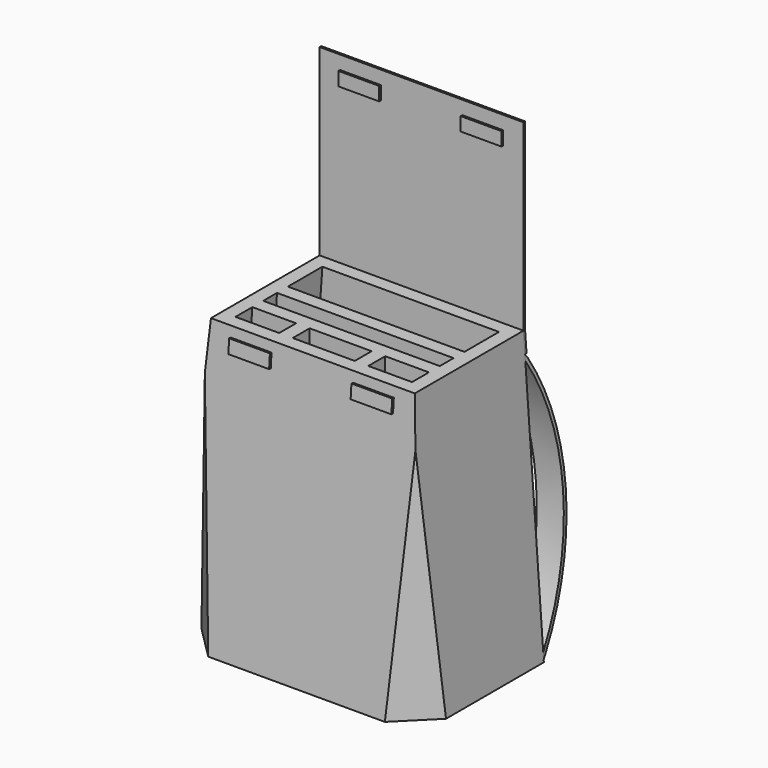
from build123d import *

# Parameters (mm, degrees)
F0_W      = 300
F0_H      = 200
F1_DEPTH  = 420
F3_DEPTH  = 420
F5_DEPTH  = 360
F7_DEPTH  = 230.001
F9_DEPTH  = 1000
F10_T     = -20
F11_W     = 317.0409461497
F11_H     = 20
F12_DEPTH = 400
F13_DEPTH = 25
F14_DEPTH = 25
F15_DEPTH = 400
F16_DEPTH = 400
F17_DEPTH = 25
F18_DEPTH = 25
F19_DEPTH = 184.1
F20_DEPTH = 240
F22_W     = 300
F22_H     = 200
F22_R     = 3.5
F22_H_2   = 70
F22_W_2   = 60
F22_H_3   = 20
F23_DEPTH = 3
F24_DEPTH = 3
F21_W     = 60
F21_H     = 20
F25_DEPTH = 3
F27_DEPTH = 40
F28_DEPTH = 4


# Not quite as in the source:
# - a pattern or mirror of a feature is missing from the dataset's text; its kind, count and spacing are read off the source's solid


with BuildPart() as f1:
    # F0 (on Top) → F1 (new body)
    with BuildSketch(Plane.XY):
        Rectangle(F0_W, F0_H)
    extrude(amount=F1_DEPTH)

    # F2 (on face) → F3 (join)
    with BuildSketch(Plane(origin=(0, 0, 0), x_dir=(1, 0, 0), z_dir=(0, 0, -1))):
        Polygon((-180, -100), (-150, -100), (-150, 100), (150, 100), (150, -100), (180, -100), (180, 130), (-180, 130), align=None)
    extrude(amount=-F3_DEPTH)

    # F4 (on face) → F5 (cut, through all)
    with BuildSketch(Plane.YZ.offset(180)):
        Polygon((-130, 0), (-100, 420), (-130, 420), align=None)
    extrude(amount=-F5_DEPTH, mode=Mode.SUBTRACT)

    # F6 (on face) → F7 (cut, through all)
    with BuildSketch(Plane(origin=(0, 100, 0), x_dir=(-1, 0, 0), z_dir=(0, 1, 0))):
        Polygon((-180, 0), (-150, 420), (-180, 420), align=None)
        Polygon((180, 420), (150, 420), (180, 0), align=None)
    extrude(amount=-F7_DEPTH, mode=Mode.SUBTRACT)

    # F8 (on face) → F9 (cut)
    with BuildSketch(Plane(origin=(0, 0, 0), x_dir=(1, 0, 0), z_dir=(0, 0, -1))):
        Polygon((-180, 80), (-130, 130), (-180, 130), align=None)
        Polygon((180, 130), (130, 130), (180, 80), align=None)
    extrude(amount=-F9_DEPTH, mode=Mode.SUBTRACT)

    # F10
    f10_openings = [f1.faces().sort_by_distance(p)[0] for p in [
        (0, 0, 420),
    ]]
    offset(amount=F10_T, openings=f10_openings)

    # F11 (on face) → F12 (join)
    with BuildSketch(Plane.XY.offset(20)):
        with Locations((0, 6.5)):
            Rectangle(F11_W, F11_H)
    extrude(amount=F12_DEPTH)

    # F13 (cut): a face of the model
    f13_faces = [f1.faces().sort_by_distance(p)[0] for p in [
        (-155.6803153832, -3.5, 380.2377923175),
    ]]
    extrude(f13_faces, amount=-F13_DEPTH, mode=Mode.SUBTRACT)

    # F14 (cut): a face of the model
    f14_faces = [f1.faces().sort_by_distance(p)[0] for p in [
        (155.6803153832, -3.5, 380.2377923175),
    ]]
    extrude(f14_faces, amount=-F14_DEPTH, mode=Mode.SUBTRACT)

    # F11 (on face) → F15 (join)
    with BuildSketch(Plane.XY.offset(20)):
        Polygon((158.5204730748, -28.9), (-158.5204730748, -28.9), (-158.5204730748, -48.9), (-65.6204730748, -48.9), (-45.6204730748, -48.9), (45.6204730748, -48.9), (65.6204730748, -48.9), (158.5204730748, -48.9), align=None)
    extrude(amount=F15_DEPTH)

    # F11 (on face) → F16 (join)
    with BuildSketch(Plane.XY.offset(20)):
        Polygon((-45.6204730748, -48.9), (-65.6204730748, -48.9), (-65.6204730748, -83.5204730748), (-65.6204730748, -108.5204730748), (-45.6204730748, -108.5204730748), (-45.6204730748, -83.5204730748), align=None)
        Polygon((65.6204730748, -83.5204730748), (65.6204730748, -48.9), (45.6204730748, -48.9), (45.6204730748, -83.5204730748), (45.6204730748, -108.5204730748), (65.6204730748, -108.5204730748), align=None)
    extrude(amount=F16_DEPTH)

    # F17 (cut): faces of the model
    f17_faces = [f1.faces().sort_by_distance(p)[0] for p in [
        (-155.6803153832, -48.9, 380.2377923175),
        (155.6803153832, -48.9, 380.2377923175),
    ]]
    extrude(f17_faces, amount=-F17_DEPTH, mode=Mode.SUBTRACT)

    # F18 (cut): faces of the model
    f18_faces = [f1.faces().sort_by_distance(p)[0] for p in [
        (-65.6204730748, -105.6803153832, 380.2377923175),
        (45.6204730748, -105.6803153832, 380.2377923175),
    ]]
    extrude(f18_faces, amount=-F18_DEPTH, mode=Mode.SUBTRACT)

    # F11 (on face) → F19 (join)
    with BuildSketch(Plane.XY.offset(20)):
        Polygon((158.5204730748, -73.1952556777), (158.5204730748, -48.9), (65.6204730748, -48.9), (65.6204730748, -83.5204730748), (65.6204730748, -108.5204730748), (123.1952556777, -108.5204730748), align=None)
    extrude(amount=F19_DEPTH)

    # F11 (on face) → F20 (join)
    with BuildSketch(Plane.XY.offset(20)):
        Polygon((45.6204730748, -48.9), (-45.6204730748, -48.9), (-45.6204730748, -83.5204730748), (-45.6204730748, -108.5204730748), (45.6204730748, -108.5204730748), (45.6204730748, -83.5204730748), align=None)
    extrude(amount=F20_DEPTH)


with BuildPart() as f23:
    # F22 (on face) → F23 (new body)
    with BuildSketch(Plane(origin=(0, 100, 0), x_dir=(-1, 0, 0), z_dir=(0, 1, 0))):
        with Locations((0, 520)):
            Rectangle(F22_W, F22_H)
        Polygon((-150, 420), (-152.1428571429, 390), (152.1428571429, 390), (150, 420), align=None)
        with Locations((-120, 405)):
            Circle(F22_R, mode=Mode.SUBTRACT)
        with Locations((0, 405)):
            Circle(F22_R, mode=Mode.SUBTRACT)
        with Locations((120, 405)):
            Circle(F22_R, mode=Mode.SUBTRACT)
        with Locations((0, 655)):
            Rectangle(F22_W, F22_H_2)
        with Locations((-90, 660)):
            Rectangle(F22_W_2, F22_H_3, mode=Mode.SUBTRACT)
        with Locations((90, 660)):
            Rectangle(F22_W_2, F22_H_3, mode=Mode.SUBTRACT)
        with Locations((-90, 660)):
            Rectangle(F22_W_2, F22_H_3)
        with Locations((90, 660)):
            Rectangle(F22_W_2, F22_H_3)
    extrude(amount=F23_DEPTH)


with BuildPart() as f24:
    # F22 (on face) → F24 (new body)
    with BuildSketch(Plane(origin=(0, 100, 0), x_dir=(-1, 0, 0), z_dir=(0, 1, 0))):
        with Locations((90, 660)):
            Rectangle(F22_W_2, F22_H_3)
    extrude(amount=-F24_DEPTH)


with BuildPart() as f24b:
    # F22 (on face) → F24, piece 2 (new body)
    with BuildSketch(Plane(origin=(0, 100, 0), x_dir=(-1, 0, 0), z_dir=(0, 1, 0))):
        with Locations((-90, 660)):
            Rectangle(F22_W_2, F22_H_3)
    extrude(amount=-F24_DEPTH)


with BuildPart() as f25:
    # F21 (on face) → F25 (new body)
    with BuildSketch(Plane(origin=(0, -129.3401015228, 9.2385786802), x_dir=(1, 0, 0), z_dir=(0, -0.9974586998, 0.07124705))):
        with Locations((-90, 386.8079489301)):
            Rectangle(F21_W, F21_H)
    extrude(amount=F25_DEPTH)


with BuildPart() as f25b:
    # F21 (on face) → F25, piece 2 (new body)
    with BuildSketch(Plane(origin=(0, -129.3401015228, 9.2385786802), x_dir=(1, 0, 0), z_dir=(0, -0.9974586998, 0.07124705))):
        with Locations((90, 386.8079489301)):
            Rectangle(F21_W, F21_H)
    extrude(amount=F25_DEPTH)


with BuildPart() as f27:
    # F26 (on face) → F27 (new body)
    with BuildSketch(Plane(origin=(179.0862944162, 0, 12.7918781726), x_dir=(0, 1, 0), z_dir=(0.9974586998, 0, 0.07124705))):
        with BuildLine():
            ThreePointArc((100, 370.1041340828), (153.0191995097, 185.0520670414), (100, 0))
            Line((100, 0), (100, -9.441984234))
            Line((100, -9.441984234), (104.241394541, -2.6477485431))
            ThreePointArc((104.241394541, -2.6477485431), (158.0191995097, 185.0520670414), (104.241394541, 372.7518826259))
            Line((104.241394541, 372.7518826259), (100, 377.5273796043))
            Line((100, 377.5273796043), (100, 370.1041340828))
        make_face()
    extrude(amount=-F27_DEPTH)


with BuildPart() as f27_copies_1:
    # F27_copies: instance of F27
    add(f27.part.mirror(Plane(origin=(0, 0, 0), x_dir=(0, 0, -1), z_dir=(-1, 0, 0))))


with BuildPart() as f28:
    # F22 (on face) → F28 (new body)
    with BuildSketch(Plane(origin=(0, 100, 0), x_dir=(-1, 0, 0), z_dir=(0, 1, 0))):
        with Locations((-120, 405)):
            Circle(F22_R)
    extrude(amount=F28_DEPTH)


with BuildPart() as f28b:
    # F22 (on face) → F28, piece 2 (new body)
    with BuildSketch(Plane(origin=(0, 100, 0), x_dir=(-1, 0, 0), z_dir=(0, 1, 0))):
        with Locations((0, 405)):
            Circle(F22_R)
    extrude(amount=F28_DEPTH)


with BuildPart() as f28c:
    # F22 (on face) → F28, piece 3 (new body)
    with BuildSketch(Plane(origin=(0, 100, 0), x_dir=(-1, 0, 0), z_dir=(0, 1, 0))):
        with Locations((120, 405)):
            Circle(F22_R)
    extrude(amount=F28_DEPTH)


solid = Compound([f1.part, f23.part, f24.part, f24b.part, f25.part, f25b.part, f27.part, f27_copies_1.part, f28.part, f28b.part, f28c.part])
